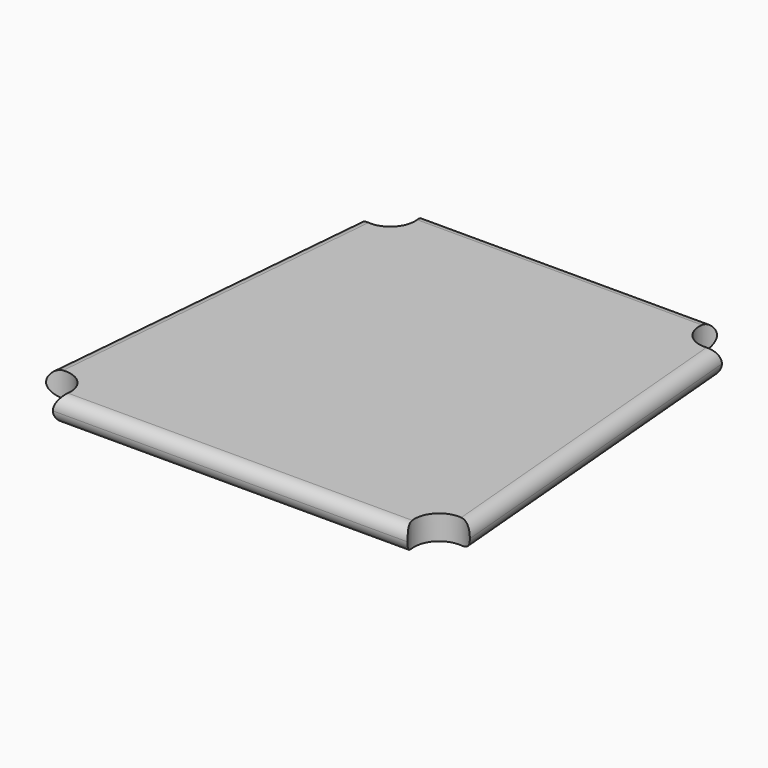
from build123d import *

# Parameters (mm, degrees)
F1_DEPTH = 25.4
F2_R     = 12.69999


# Not quite as in the source:
# - a fillet or chamfer is up to 0.001 mm smaller than in the source, because OpenCascade refuses the exact size


with BuildPart() as f1:
    # F0 (on Top) → F1 (new body)
    with BuildSketch(Plane.XY):
        with BuildLine():
            ThreePointArc((-219.075, -183.3721313551), (-185.1905403178, -185.2885689585), (-183.4590722629, -219.182983829))
            Line((-183.4590722629, -219.182983829), (183.4590722629, -219.182983829))
            ThreePointArc((183.4590722629, -219.182983829), (185.1905403178, -185.2885689585), (219.075, -183.3721313551))
            Line((219.075, -183.3721313551), (187.072348327, 182.4198510941))
            ThreePointArc((187.072348327, 182.4198510941), (153.9534082329, 185.8090843811), (152.6381313551, 219.075))
            Line((152.6381313551, 219.075), (-152.6381313551, 219.075))
            ThreePointArc((-152.6381313551, 219.075), (-153.9534082329, 185.8090843811), (-187.072348327, 182.4198510941))
            Line((-187.072348327, 182.4198510941), (-219.075, -183.3721313551))
        make_face()
    extrude(amount=F1_DEPTH)

    # F2 (radius 12.7 in the source; OpenCascade refuses exactly that, so slightly less here)
    f2_edges = [f1.edges().sort_by_distance(p)[0] for p in [
        (-203.073674, -0.47614, 25.4),
        (0, 219.075, 25.4),
        (0, -219.182984, 25.4),
        (203.073674, -0.47614, 25.4),
        (-203.073674, -0.47614, 0),
        (0, -219.182984, 0),
        (0, 219.075, 0),
        (203.073674, -0.47614, 0),
    ]]
    fillet(f2_edges, radius=F2_R)


solid = f1.part
